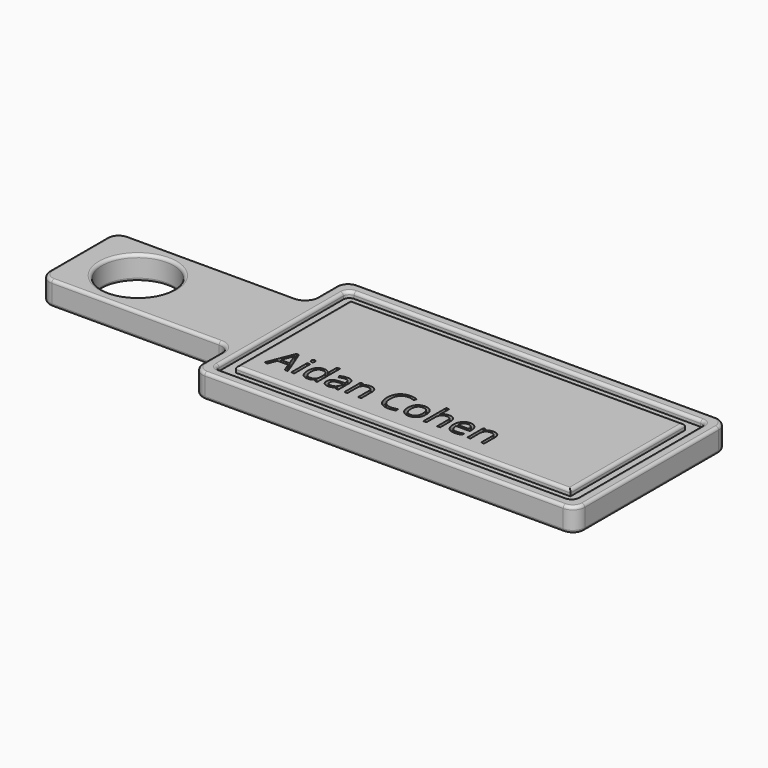
from build123d import *

# Parameters (mm, degrees)
F0_W          = 203.2
F0_H          = 101.6
F1_DEPTH      = 25.4
F2_R          = 38.1
F3_DEPTH      = 25.4
F6_DEPTH      = 6.35
F7_R          = 6.35
F8_R          = 12.7
F9_R          = 3.175
F10_TEXT_SIZE = 39.7980057945
F11_DEPTH     = 5.08


# Not quite as in the source:
# - Text() gives the source's letters only with a copy of the font that has no kerning and outlines rounded to 1/6400 em; it was checked with that copy


with BuildPart() as f1:
    # F0 (on Top) → F1 (new body)
    with BuildSketch(Plane.XY):
        Polygon((0, 50.8), (0, 0), (406.4, 0), (406.4, 203.2), (0, 203.2), (0, 152.4), align=None)
        with Locations((-101.6, 101.6)):
            Rectangle(F0_W, F0_H)
    extrude(amount=F1_DEPTH)

    # F2 (on face) → F3 (cut)
    with BuildSketch(Plane.XY.offset(25.4)):
        with Locations((-139.7, 101.6)):
            Circle(F2_R)
    extrude(amount=-F3_DEPTH, mode=Mode.SUBTRACT)

    # F5 (on face) → F6 (cut)
    with BuildSketch(Plane.XY.offset(25.4)):
        Polygon((12.6999939203, 50.8), (12.6999939203, 12.6999939203), (393.7000060797, 12.6999939203), (393.7000060797, 190.5000060797), (12.6999939203, 190.5000060797), (12.6999939203, 152.4), align=None)
        Polygon((25.4000002861, 50.8), (25.4000002861, 152.4), (25.4000002861, 177.7999997139), (380.9999997139, 177.7999997139), (380.9999997139, 25.4000002861), (25.4000002861, 25.4000002861), align=None, mode=Mode.SUBTRACT)
    extrude(amount=-F6_DEPTH, mode=Mode.SUBTRACT)

    # F7
    f7_edges = [f1.edges().sort_by_distance(p)[0] for p in [
        (12.699994, 12.699994, 22.225),
        (12.699994, 190.500006, 22.225),
        (393.700006, 190.500006, 22.225),
        (393.700006, 12.699994, 22.225),
    ]]
    fillet(f7_edges, radius=F7_R)

    # F8
    f8_edges = [f1.edges().sort_by_distance(p)[0] for p in [
        (406.4, 0, 12.7),
        (0, 0, 12.7),
        (-203.2, 50.8, 12.7),
        (0, 50.8, 12.7),
        (-203.2, 152.4, 12.7),
        (0, 203.2, 12.7),
        (406.4, 203.2, 12.7),
        (0, 152.4, 12.7),
    ]]
    fillet(f8_edges, radius=F8_R)

    # F9
    f9_edges = [f1.edges().sort_by_distance(p)[0] for p in [
        (203.2, 177.8, 25.4),
        (381, 101.6, 25.4),
        (203.2, 25.4, 25.4),
        (25.4, 101.6, 25.4),
        (0, 25.4, 25.4),
        (-3.719744, 47.080256, 25.4),
        (3.719744, 3.719744, 25.4),
        (-101.6, 50.8, 25.4),
        (203.2, 0, 25.4),
        (-199.480256, 54.519744, 25.4),
        (402.680256, 3.719744, 25.4),
        (-203.2, 101.6, 25.4),
        (406.4, 101.6, 25.4),
        (-199.480256, 148.680256, 25.4),
        (402.680256, 199.480256, 25.4),
        (-101.6, 152.4, 25.4),
        (203.2, 203.2, 25.4),
        (-3.719744, 156.119744, 25.4),
        (3.719744, 199.480256, 25.4),
        (0, 177.8, 25.4),
        (203.2, 12.699994, 25.4),
        (14.559866, 14.559866, 25.4),
        (391.840134, 14.559866, 25.4),
        (12.699994, 101.6, 25.4),
        (393.700006, 101.6, 25.4),
        (14.559866, 188.640134, 25.4),
        (391.840134, 188.640134, 25.4),
        (203.2, 190.500006, 25.4),
        (-177.8, 101.6, 25.4),
        (0, 25.4, 0),
        (-3.719744, 47.080256, 0),
        (3.719744, 3.719744, 0),
        (-101.6, 50.8, 0),
        (203.2, 0, 0),
        (-199.480256, 54.519744, 0),
        (402.680256, 3.719744, 0),
        (-203.2, 101.6, 0),
        (406.4, 101.6, 0),
        (-199.480256, 148.680256, 0),
        (402.680256, 199.480256, 0),
        (-101.6, 152.4, 0),
        (203.2, 203.2, 0),
        (-3.719744, 156.119744, 0),
        (3.719744, 199.480256, 0),
        (0, 177.8, 0),
        (-177.8, 101.6, 0),
    ]]
    fillet(f9_edges, radius=F9_R)

    # F10 (on face) → F11 (cut)
    with BuildSketch(Plane.XY.offset(25.4)):
        with Locations((39.762057364, 45.2535934746)):
            Text('Aidan Cohen', F10_TEXT_SIZE, font='Open Sans', text_align=(TextAlign.LEFT, TextAlign.BOTTOM))
    extrude(amount=-F11_DEPTH, mode=Mode.SUBTRACT)


solid = f1.part
